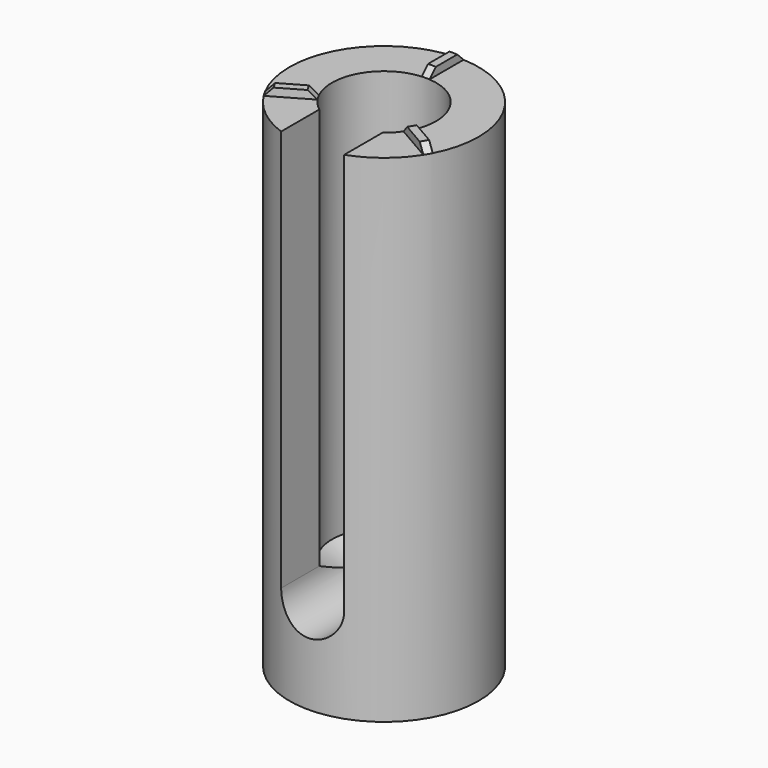
from build123d import *

# Parameters (mm, degrees)
F0_R      = 9.525
F1_DEPTH  = 50.8
F3_D      = 10.4902
F3_DEPTH  = 41.275
F3_TIP    = 3.1515740329
F5_D      = 3.4544
F7_DEPTH  = 0.79375
F8_SIZE   = 0.79375
F10_DEPTH = 25.4


with BuildPart() as f1:
    # F0 (on Top) → F1 (new body)
    with BuildSketch(Plane.XY):
        Circle(F0_R)
    extrude(amount=F1_DEPTH)

    # F3
    with Locations(Plane.XY.offset(50.8)):
        with Locations((0, 0)):
            Hole(F3_D / 2, depth=F3_DEPTH)
            with Locations((0, 0, -(F3_DEPTH + F3_TIP / 2))):  # 118° drill point
                Cone(0, F3_D / 2, F3_TIP, mode=Mode.SUBTRACT)

    # F5 (through all)
    with Locations(Plane(origin=(0, 0, 0), x_dir=(1, 0, 0), z_dir=(0, 0, -1))):
        with Locations((0, 0)):
            Hole(F5_D / 2)

    # F6 (on face) → F7 (cut)
    with BuildSketch(Plane.XY.offset(50.8)):
        with BuildLine():
            ThreePointArc((-4.7278053569, -2.2713279193), (-4.5423898454, 2.62255), (-0.396875, 5.2300635029))
            Line((-0.396875, 5.2300635029), (-0.396875, 9.5167281791))
            ThreePointArc((-0.396875, 9.5167281791), (-8.248891971, 4.7625), (-8.440165864, -4.4146602574))
            Line((-8.440165864, -4.4146602574), (-4.7278053569, -2.2713279193))
        make_face()
        with BuildLine():
            Line((8.043290864, -5.1020679217), (4.3309303569, -2.9587355836))
            ThreePointArc((4.3309303569, -2.9587355836), (0, -5.2451), (-4.3309303569, -2.9587355836))
            Line((-4.3309303569, -2.9587355836), (-8.043290864, -5.1020679217))
            ThreePointArc((-8.043290864, -5.1020679217), (0, -9.525), (8.043290864, -5.1020679217))
        make_face()
        with BuildLine():
            ThreePointArc((0.396875, 5.2300635029), (3.8466038965, 3.5657695486), (5.2451, 0))
            ThreePointArc((5.2451, 0), (5.1141414669, -1.1647450649), (4.7278053569, -2.2713279193))
            Line((4.7278053569, -2.2713279193), (8.440165864, -4.4146602574))
            ThreePointArc((8.440165864, -4.4146602574), (9.2498163456, -2.2729985862), (9.525, 0))
            ThreePointArc((9.525, 0), (6.8740766425, 6.5933826912), (0.396875, 9.5167281791))
            Line((0.396875, 9.5167281791), (0.396875, 5.2300635029))
        make_face()
    extrude(amount=-F7_DEPTH, mode=Mode.SUBTRACT)

    # F8
    f8_edges = [f1.edges().sort_by_distance(p)[0] for p in [
        (8.248892, -4.7625, 50.8),
        (0, 9.525, 50.8),
        (-8.248892, -4.7625, 50.8),
        (4.54239, -2.62255, 50.8),
        (-4.54239, -2.62255, 50.8),
        (0, 5.2451, 50.8),
    ]]
    chamfer(f8_edges, length=F8_SIZE)

    # F9 (on Front) → F10 (cut)
    with BuildSketch(Plane.XZ):
        with BuildLine():
            ThreePointArc((3.175, 52.54625), (0, 55.72125), (-3.175, 52.54625))
            Line((-3.175, 52.54625), (-3.175, 9.525))
            ThreePointArc((-3.175, 9.525), (0, 6.35), (3.175, 9.525))
            Line((3.175, 9.525), (3.175, 52.54625))
        make_face()
    extrude(amount=F10_DEPTH, mode=Mode.SUBTRACT)


solid = f1.part
